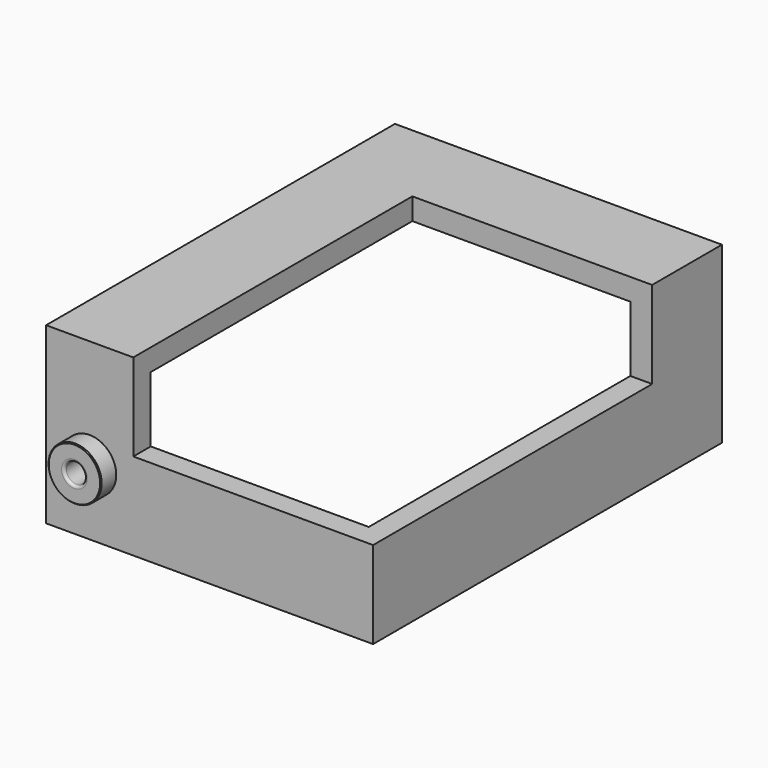
from build123d import *

# Parameters (mm, degrees)
F1_DEPTH      = 12.7
F1_DEPTH_BACK = 12.7
F3_DEPTH      = 25.4
F5_DEPTH      = 25.4
F6_R          = 6.35
F7_DEPTH      = 6.35
F8_R          = 6.35
F8_R_2        = 2.9718
F9_DEPTH      = 6.35
F10_R         = 7.7390625
F10_R_2       = 2.9718
F11_DEPTH     = 5.55625
F12_R         = 0.762
F13_SIZE      = 0.254


with BuildPart() as f1:
    # F0 (on Right) → F1 (new body, two sides)
    with BuildSketch(Plane.YZ) as f1_sk:
        Polygon((120.65, 25.4), (120.65, 31.75), (-6.35, 31.75), (-6.35, -19.05), (0, -19.05), (0, 25.4), align=None)
    extrude(amount=F1_DEPTH)
    extrude(f1_sk.sketch, amount=-F1_DEPTH_BACK)

    # F2 (on face) → F3 (join)
    with BuildSketch(Plane(origin=(0, 0, -19.05), x_dir=(1, 0, 0), z_dir=(0, 0, -1))):
        Polygon((12.7, 6.35), (12.7, 0), (76.2, 0), (76.2, -120.65), (82.55, -120.65), (82.55, 6.35), align=None)
    extrude(amount=-F3_DEPTH)

    # F4 (on face) → F5 (join)
    with BuildSketch(Plane(origin=(0, 120.65, 0), x_dir=(-1, 0, 0), z_dir=(0, 1, 0))):
        Polygon((-12.7, 25.4), (-12.7, 31.75), (-82.55, 31.75), (-82.55, 6.35), (-76.2, 6.35), (-76.2, 25.4), align=None)
    extrude(amount=-F5_DEPTH)

    # F6 (on face) → F7 (cut, through all)
    with BuildSketch(Plane.XZ.offset(6.35)):
        Circle(F6_R)
    extrude(amount=-F7_DEPTH, mode=Mode.SUBTRACT)


with BuildPart() as f9:
    # F8 (on face) → F9 (new body)
    with BuildSketch(Plane.XZ.offset(6.35)):
        Circle(F8_R)
        Circle(F8_R_2, mode=Mode.SUBTRACT)
    extrude(amount=-F9_DEPTH)

    # F10 (on face) → F11 (join)
    with BuildSketch(Plane.XZ.offset(6.35)):
        Circle(F10_R)
        Circle(F10_R_2, mode=Mode.SUBTRACT)
    extrude(amount=F11_DEPTH)

    # F12
    f12_edges = [f9.edges().sort_by_distance(p)[0] for p in [
        (-2.9718, -11.90625, 0),
    ]]
    fillet(f12_edges, radius=F12_R)

    # F13
    f13_edges = [f9.edges().sort_by_distance(p)[0] for p in [
        (-7.739063, -11.90625, 0),
    ]]
    chamfer(f13_edges, length=F13_SIZE)


solid = Compound([f1.part, f9.part])
